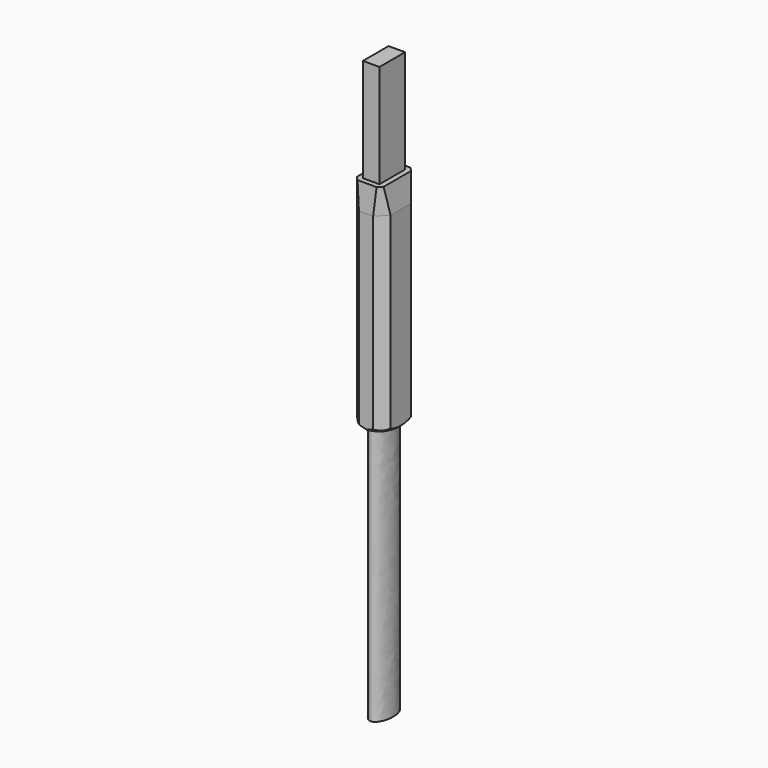
from build123d import *

# Parameters (mm, degrees)
F1_DEPTH      = 93.98
F5_W          = 8.128
F5_H          = 15.748
F6_DEPTH      = 50.8
F8_DEPTH      = 127
F9_SIZE       = 0.8382
F10_SIZE      = 0.381
F11_T4_DEPTH  = 25.5498757067
F11_T9_DEPTH  = 25.5498757067
F11_T14_DEPTH = 25.5498757067
F11_T19_DEPTH = 25.5498757067
F11_T24_DEPTH = 25.5498757067
F11_T29_DEPTH = 25.5498757067
F11_T34_DEPTH = 25.5498757067
F11_T39_DEPTH = 25.5498757067


# Not quite as in the source:
# - a fillet or chamfer that OpenCascade refuses, or shapes differently, is made with other operations: its cross-section is extruded or revolved along the edge and cut away or added


with BuildPart() as f1:
    # F0 (on Top) → F1 (new body)
    with BuildSketch(Plane.XY):
        Polygon((-8.255, -6.2930149161), (-3.4990149161, -11.049), (3.4990149161, -11.049), (8.255, -6.2930149161), (8.255, 6.2930149161), (3.4990149161, 11.049), (-3.4990149161, 11.049), (-8.255, 6.2930149161), align=None)
    extrude(amount=F1_DEPTH)

    # F3 (on offset) → F4 section 0
    with BuildSketch(Plane.XY.offset(106.68)):
        Polygon((-6.604, -8.4828302834), (-4.6728302834, -10.414), (4.6728302834, -10.414), (6.604, -8.4828302834), (6.604, 8.4828302834), (4.6728302834, 10.414), (-4.6728302834, 10.414), (-6.604, 8.4828302834), align=None)
    # F1_face (on face) → F4 section 1
    with BuildSketch(Plane.XY.offset(93.98)):
        Polygon((-8.255, 6.2930149161), (-8.255, -6.2930149161), (-3.4990149161, -11.049), (3.4990149161, -11.049), (8.255, -6.2930149161), (8.255, 6.2930149161), (3.4990149161, 11.049), (-3.4990149161, 11.049), align=None)
    loft()

    # F5 (on face) → F6 (join)
    with BuildSketch(Plane.XY.offset(106.68)):
        Rectangle(F5_W, F5_H)
    extrude(amount=F6_DEPTH)

    # F7 (on face) → F8 (join)
    with BuildSketch(Plane(origin=(0, 0, 0), x_dir=(1, 0, 0), z_dir=(0, 0, -1))):
        with BuildLine():
            add(Edge.make_bspline(
                [(0, 8.255), (-7.6989658396, 8.255), (-3.8494829198, -4.1275), (0, -16.51), (3.8494829198, -4.1275), (7.6989658396, 8.255), (0, 8.255)],
                knots=[0, 0, 0, 2.0943951024, 2.0943951024, 4.1887902048, 4.1887902048, 6.2831853072, 6.2831853072, 6.2831853072], degree=2, weights=[1, 0.5, 1, 0.5, 1, 0.5, 1]))
        make_face()
    extrude(amount=F8_DEPTH)

    # F9
    f9_edges = [f1.edges().sort_by_distance(p)[0] for p in [
        (-5.877007, -8.671007, 0),
        (5.877007, -8.671007, 0),
        (-5.877007, 8.671007, 0),
        (5.877007, 8.671007, 0),
    ]]
    chamfer(f9_edges, length=F9_SIZE)

    # F10
    f10_edges = [f1.edges().sort_by_distance(p)[0] for p in [
        (0, -11.049, 0),
        (-8.255, 0, 0),
        (0, 11.049, 0),
        (8.255, 0, 0),
    ]]
    chamfer(f10_edges, length=F10_SIZE)

    # F11: fillet of radius 17.78 on 8 edges, made by hand


with BuildPart() as f11_tool2:
    # F11_s3 → F11_t4 (new body)
    with BuildSketch(Plane(origin=(-13.5324141085, -5.6053094554, 13.5324141085), x_dir=(-0.3826834324, 0.9238795325, 0), z_dir=(0.6785983445, 0.2810846377, -0.6785983445))):
        with BuildLine():
            ThreePointArc((2.7536579732, -5.0095172844), (-2.0575753571, -5.6728460589), (-6.8688086874, -5.0095172844))
            Line((-6.8688086874, -5.0095172844), (-2.0575753571, -6.361881062))
            Line((-2.0575753571, -6.361881062), (2.7536579732, -5.0095172844))
        make_face()
    extrude(amount=F11_T4_DEPTH)

    split(bisect_by=Plane.XY, keep=Keep.TOP)


with BuildPart() as f1_1:
    add(f1.part)

    # F11_t1: cut F11_tool2
    add(f11_tool2.part, mode=Mode.SUBTRACT)


with BuildPart() as f11_tool7:
    # F11_s8 → F11_t9 (new body)
    with BuildSketch(Plane(origin=(1.2641805217, 3.0520017608, -3.0520017608), x_dir=(0.9238795325, -0.3826834324, 0), z_dir=(-0.2810846377, -0.6785983445, 0.6785983445))):
        with BuildLine():
            ThreePointArc((-3.2182717635, -6.0356271331), (1.5929615668, -6.6989559076), (6.4041948971, -6.0356271331))
            Line((6.4041948971, -6.0356271331), (1.5929615668, -7.3879909107))
            Line((1.5929615668, -7.3879909107), (-3.2182717635, -6.0356271331))
        make_face()
    extrude(amount=F11_T9_DEPTH)

    split(bisect_by=Plane.XY, keep=Keep.TOP)


with BuildPart() as f1_2:
    add(f1_1.part)

    # F11_t6: cut F11_tool7
    add(f11_tool7.part, mode=Mode.SUBTRACT)


with BuildPart() as f11_tool12:
    # F11_s13 → F11_t14 (new body)
    with BuildSketch(Plane(origin=(-1.2641805217, 3.0520017608, -3.0520017608), x_dir=(0.9238795325, 0.3826834324, 0), z_dir=(0.2810846377, -0.6785983445, 0.6785983445))):
        with BuildLine():
            ThreePointArc((-6.4041948971, -6.0356271331), (-1.5929615668, -6.6989559076), (3.2182717635, -6.0356271331))
            Line((3.2182717635, -6.0356271331), (-1.5929615668, -7.3879909107))
            Line((-1.5929615668, -7.3879909107), (-6.4041948971, -6.0356271331))
        make_face()
    extrude(amount=F11_T14_DEPTH)

    split(bisect_by=Plane.XY, keep=Keep.TOP)


with BuildPart() as f1_3:
    add(f1_2.part)

    # F11_t11: cut F11_tool12
    add(f11_tool12.part, mode=Mode.SUBTRACT)


with BuildPart() as f11_tool17:
    # F11_s18 → F11_t19 (new body)
    with BuildSketch(Plane(origin=(-3.8056892495, 1.5763681013, -3.8056892495), x_dir=(0.3826834324, 0.9238795325, 0), z_dir=(0.6785983445, -0.2810846377, 0.6785983445))):
        with BuildLine():
            ThreePointArc((2.7536579732, -5.0095172844), (-2.0575753571, -5.6728460589), (-6.8688086874, -5.0095172844))
            Line((-6.8688086874, -5.0095172844), (-2.0575753571, -6.361881062))
            Line((-2.0575753571, -6.361881062), (2.7536579732, -5.0095172844))
        make_face()
    extrude(amount=F11_T19_DEPTH)

    split(bisect_by=Plane.XY, keep=Keep.TOP)


with BuildPart() as f1_4:
    add(f1_3.part)

    # F11_t16: cut F11_tool17
    add(f11_tool17.part, mode=Mode.SUBTRACT)


with BuildPart() as f11_tool22:
    # F11_s23 → F11_t24 (new body)
    with BuildSketch(Plane(origin=(-3.8056892495, -1.5763681013, -3.8056892495), x_dir=(-0.3826834324, 0.9238795325, 0), z_dir=(0.6785983445, 0.2810846377, 0.6785983445))):
        with BuildLine():
            ThreePointArc((6.8688086874, -5.0095172844), (2.0575753571, -5.6728460589), (-2.7536579732, -5.0095172844))
            Line((-2.7536579732, -5.0095172844), (2.0575753571, -6.361881062))
            Line((2.0575753571, -6.361881062), (6.8688086874, -5.0095172844))
        make_face()
    extrude(amount=F11_T24_DEPTH)

    split(bisect_by=Plane.XY, keep=Keep.TOP)


with BuildPart() as f1_5:
    add(f1_4.part)

    # F11_t21: cut F11_tool22
    add(f11_tool22.part, mode=Mode.SUBTRACT)


with BuildPart() as f11_tool27:
    # F11_s28 → F11_t29 (new body)
    with BuildSketch(Plane(origin=(-1.2641805217, -3.0520017608, -3.0520017608), x_dir=(-0.9238795325, 0.3826834324, 0), z_dir=(0.2810846377, 0.6785983445, 0.6785983445))):
        with BuildLine():
            ThreePointArc((6.4041948971, -6.0356271331), (1.5929615668, -6.6989559076), (-3.2182717635, -6.0356271331))
            Line((-3.2182717635, -6.0356271331), (1.5929615668, -7.3879909107))
            Line((1.5929615668, -7.3879909107), (6.4041948971, -6.0356271331))
        make_face()
    extrude(amount=F11_T29_DEPTH)

    split(bisect_by=Plane.XY, keep=Keep.TOP)


with BuildPart() as f1_6:
    add(f1_5.part)

    # F11_t26: cut F11_tool27
    add(f11_tool27.part, mode=Mode.SUBTRACT)


with BuildPart() as f11_tool32:
    # F11_s33 → F11_t34 (new body)
    with BuildSketch(Plane(origin=(1.2641805217, -3.0520017608, -3.0520017608), x_dir=(-0.9238795325, -0.3826834324, 0), z_dir=(-0.2810846377, 0.6785983445, 0.6785983445))):
        with BuildLine():
            ThreePointArc((3.2182717635, -6.0356271331), (-1.5929615668, -6.6989559076), (-6.4041948971, -6.0356271331))
            Line((-6.4041948971, -6.0356271331), (-1.5929615668, -7.3879909107))
            Line((-1.5929615668, -7.3879909107), (3.2182717635, -6.0356271331))
        make_face()
    extrude(amount=F11_T34_DEPTH)

    split(bisect_by=Plane.XY, keep=Keep.TOP)


with BuildPart() as f1_7:
    add(f1_6.part)

    # F11_t31: cut F11_tool32
    add(f11_tool32.part, mode=Mode.SUBTRACT)


with BuildPart() as f11_tool37:
    # F11_s38 → F11_t39 (new body)
    with BuildSketch(Plane(origin=(-13.5324141085, 5.6053094554, 13.5324141085), x_dir=(0.3826834324, 0.9238795325, 0), z_dir=(0.6785983445, -0.2810846377, -0.6785983445))):
        with BuildLine():
            ThreePointArc((6.8688086874, -5.0095172844), (2.0575753571, -5.6728460589), (-2.7536579732, -5.0095172844))
            Line((-2.7536579732, -5.0095172844), (2.0575753571, -6.361881062))
            Line((2.0575753571, -6.361881062), (6.8688086874, -5.0095172844))
        make_face()
    extrude(amount=F11_T39_DEPTH)

    split(bisect_by=Plane.XY, keep=Keep.TOP)


with BuildPart() as f1_8:
    add(f1_7.part)

    # F11_t36: cut F11_tool37
    add(f11_tool37.part, mode=Mode.SUBTRACT)


solid = f1_8.part
